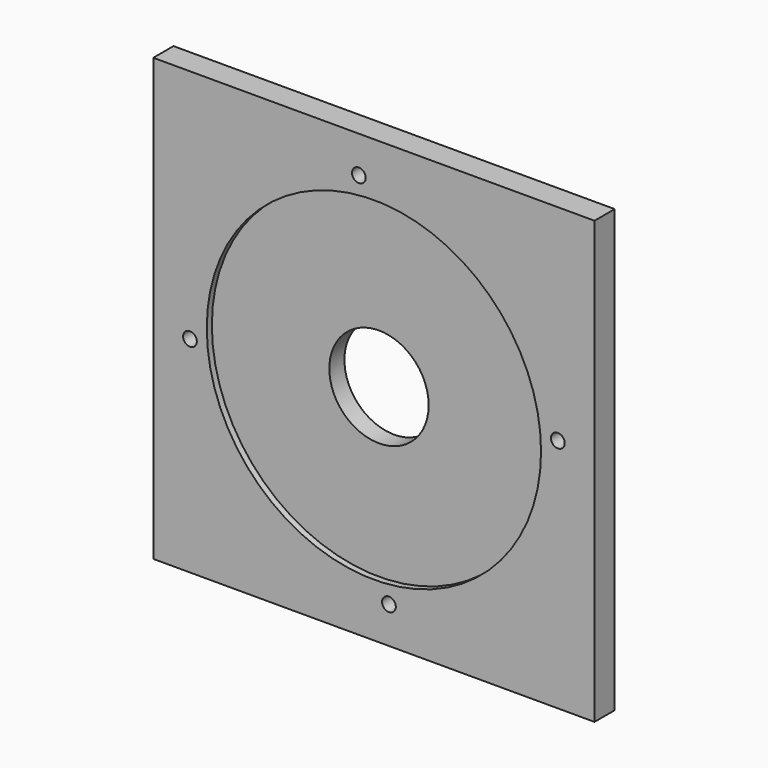
from build123d import *

# Parameters (mm, degrees)
F0_W     = 110.99
F0_H     = 110.99
F0_R     = 1.727
F0_R_2   = 12.5
F1_DEPTH = 6.35
F2_R     = 42.045
F3_DEPTH = 1.6


# Not quite as in the source:
# - a feature names something its author has since deleted; it is built from what else it names


with BuildPart() as f1:
    # F0 (on Front) → F1 (new body)
    with BuildSketch(Plane.XZ):
        Rectangle(F0_W, F0_H)
        with Locations((-46.2755883255, -3.7834937726)):
            Circle(F0_R, mode=Mode.SUBTRACT)
        with Locations((3.7834937726, -46.2755883255)):
            Circle(F0_R, mode=Mode.SUBTRACT)
        with Locations((-3.7834937726, 46.2755883255)):
            Circle(F0_R, mode=Mode.SUBTRACT)
        Circle(F0_R_2, mode=Mode.SUBTRACT)
        with Locations((46.2755883255, 3.7834937726)):
            Circle(F0_R, mode=Mode.SUBTRACT)
    extrude(amount=F1_DEPTH)

    # F2 (on face) → F3 (cut)
    with BuildSketch(Plane.XZ.offset(6.35)):
        Circle(F2_R)
    extrude(amount=-F3_DEPTH, mode=Mode.SUBTRACT)


solid = f1.part
